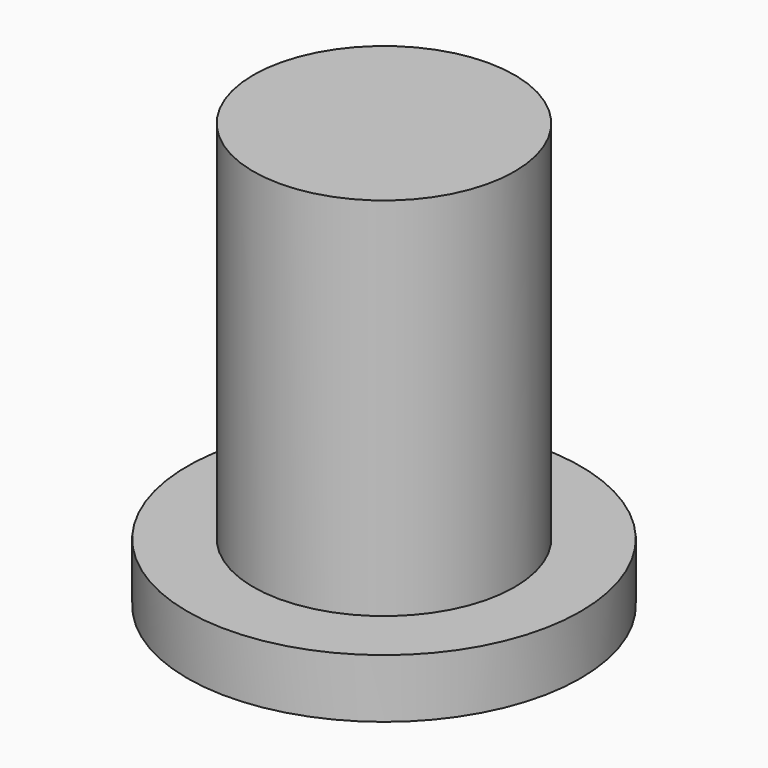
from build123d import *

# Parameters (mm, degrees)
F0_R         = 2
F1_DEPTH     = 5.6
F2_R         = 3.01
F2_R_2       = 2
F3_DEPTH     = 0.9
F4_TEXT_SIZE = 5.7946314448
F5_DEPTH     = 0.1


# Not quite as in the source:
# - Text() gives the source's letters only with a copy of the font that has no kerning and outlines rounded to 1/6400 em; it was checked with that copy


with BuildPart() as f1:
    # F0 (on Top) → F1 (new body)
    with BuildSketch(Plane.XY):
        Circle(F0_R)
    extrude(amount=F1_DEPTH)

    # F2 (on face) → F3 (join)
    with BuildSketch(Plane(origin=(0, 0, 0), x_dir=(1, 0, 0), z_dir=(0, 0, -1))):
        Circle(F2_R)
        Circle(F2_R_2, mode=Mode.SUBTRACT)
        Circle(F2_R_2)
    extrude(amount=F3_DEPTH)

    # F4 (on face) → F5 (cut)
    with BuildSketch(Plane(origin=(0, 0, -0.9), x_dir=(1, 0, 0), z_dir=(0, 0, -1))):
        with Locations((-1.2109874308, -2.0860673201)):
            Text('I', F4_TEXT_SIZE, font='Tinos', font_style=FontStyle.BOLD, text_align=(TextAlign.LEFT, TextAlign.BOTTOM))
    extrude(amount=-F5_DEPTH, mode=Mode.SUBTRACT)


solid = f1.part
